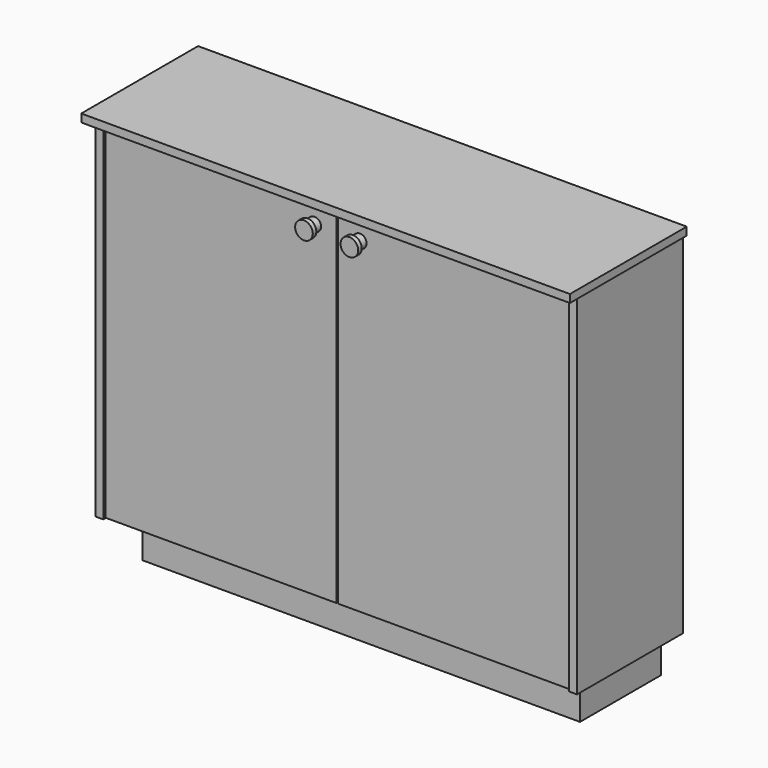
from build123d import *

# Parameters (mm, degrees)
F0_W      = 1020
F0_H      = 17.9999992251
F1_DEPTH  = 280
F2_DEPTH  = 280
F3_W      = 280
F3_H      = 795.9999984503
F4_DEPTH  = 18
F5_W      = 280
F5_H      = 795.9999984503
F6_DEPTH  = 18
F7_W      = 1091.9999984503
F7_H      = 280
F8_DEPTH  = 18
F9_W      = 18
F9_H      = 795.9999984503
F10_DEPTH = 21
F11_DEPTH = 21
F12_DEPTH = 21
F14_DEPTH = 100
F15_W     = 508.5
F15_H     = 760
F16_DEPTH = 18
F17_DEPTH = 18
F18_R     = 15
F19_DEPTH = 30
F20_R     = 20
F20_R_2   = 15
F21_DEPTH = 10


with BuildPart() as f1:
    # F0 (on Front) → F1 (new body)
    with BuildSketch(Plane.XZ):
        with Locations((0, 388.9999996126)):
            Rectangle(F0_W, F0_H)
    extrude(amount=-F1_DEPTH)

    # F0 (on Front) → F2 (join)
    with BuildSketch(Plane.XZ):
        Polygon((510, -397.9999992251), (527.9999992251, -397.9999992251), (527.9999992251, 397.9999992251), (510, 397.9999992251), (510, 380), (510, -380), align=None)
        with Locations((0, -388.9999996126)):
            Rectangle(F0_W, F0_H)
        Polygon((-527.9999992251, -397.9999992251), (-510, -397.9999992251), (-510, -380), (-510, 380), (-510, 397.9999992251), (-527.9999992251, 397.9999992251), align=None)
        with Locations((0, 388.9999996126)):
            Rectangle(F0_W, F0_H)
    extrude(amount=-F2_DEPTH)

    # F3 (on face) → F4 (join)
    with BuildSketch(Plane.YZ.offset(527.9999992251)):
        with Locations((140, 0)):
            Rectangle(F3_W, F3_H)
    extrude(amount=F4_DEPTH)

    # F5 (on face) → F6 (join)
    with BuildSketch(Plane(origin=(-527.9999992251, 0, 0), x_dir=(0, -1, 0), z_dir=(-1, 0, 0))):
        with Locations((-140, 0)):
            Rectangle(F5_W, F5_H)
    extrude(amount=F6_DEPTH)

    # F7 (on face) → F8 (join)
    with BuildSketch(Plane.XY.offset(397.9999992251)):
        with Locations((0, 140)):
            Rectangle(F7_W, F7_H)
        Polygon((553.9999992251, 280), (545.9999992251, 280), (545.9999992251, 0), (-545.9999992251, 0), (-545.9999992251, -30), (553.9999992251, -30), align=None)
    extrude(amount=F8_DEPTH)

    # F9 (on face) → F10 (join)
    with BuildSketch(Plane.XZ):
        with Locations((-536.9999992251, 0)):
            Rectangle(F9_W, F9_H)
    extrude(amount=F10_DEPTH)

    # F9 (on face) → F11 (join)
    with BuildSketch(Plane.XZ):
        with Locations((536.9999992251, 0)):
            Rectangle(F9_W, F9_H)
    extrude(amount=F11_DEPTH)

    # F12 (add): a face of the model
    f12_faces = [f1.faces().sort_by_distance(p)[0] for p in [
        (4, -30, 406.9999992251),
    ]]
    extrude(f12_faces, amount=F12_DEPTH)

    # F13 (on face) → F14 (join)
    with BuildSketch(Plane(origin=(0, 0, -397.9999992251), x_dir=(1, 0, 0), z_dir=(0, 0, -1))):
        Polygon((-495.9999992251, -50), (-495.9999992251, -280), (-476.9999992251, -280), (-476.9999992251, -69), (476.9999992251, -69), (476.9999992251, -280), (495.9999992251, -280), (495.9999992251, -50), align=None)
    extrude(amount=F14_DEPTH)

    # F15 (on face) → F16 (join)
    with BuildSketch(Plane.XZ):
        Polygon((-1.5, 380), (-1.5, 394.9999992251), (-524.9999992251, 394.9999992251), (-524.9999992251, -394.9999992251), (-1.5, -394.9999992251), (-1.5, -380), (-510, -380), (-510, 380), align=None)
        with Locations((-255.75, 0)):
            Rectangle(F15_W, F15_H)
    extrude(amount=F16_DEPTH)

    # F15 (on face) → F17 (join)
    with BuildSketch(Plane.XZ):
        Polygon((524.9999992251, -394.9999992251), (524.9999992251, 394.9999992251), (1.5, 394.9999992251), (1.5, 380), (510, 380), (510, -380), (1.5, -380), (1.5, -394.9999992251), align=None)
        with Locations((255.75, 0)):
            Rectangle(F15_W, F15_H)
    extrude(amount=F17_DEPTH)

    # F18 (on face) → F19 (join)
    with BuildSketch(Plane.XZ.offset(18)):
        with Locations((-51.5, 344.9999992251)):
            Circle(F18_R)
    extrude(amount=F19_DEPTH)

    # F20 (on face) → F21 (join)
    with BuildSketch(Plane.XZ.offset(48)):
        with Locations((-51.5, 344.9999992251)):
            Circle(F20_R)
        with Locations((-51.5, 344.9999992251)):
            Circle(F20_R_2, mode=Mode.SUBTRACT)
    extrude(amount=-F21_DEPTH)

    # F22: F1 across plane


with BuildPart() as f1_1:
    add(f1.part)
    add(f1.part.mirror(Plane.YZ))


solid = f1_1.part
